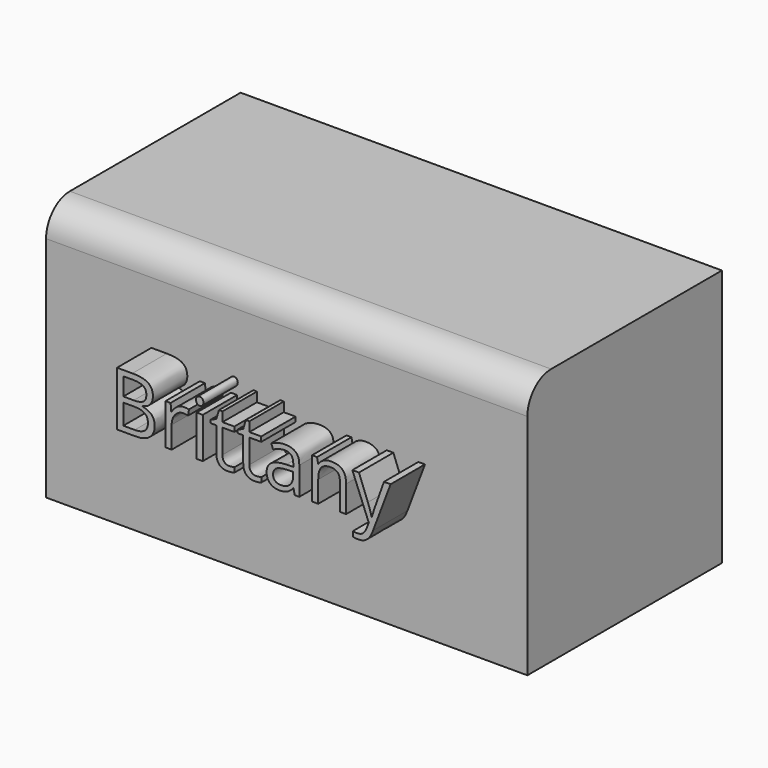
from build123d import *

# Parameters (mm, degrees)
F0_W         = 82.4485719204
F0_H         = 44.124007225
F1_DEPTH     = 41.656
F2_T         = -2.54
F3_R         = 5.08
F4_TEXT_SIZE = 13.0546641433
F5_DEPTH     = 49.022


# Not quite as in the source:
# - Text() gives the source's letters only with a copy of the font that has no kerning and outlines rounded to 1/6400 em; it was checked with that copy


with BuildPart() as f1:
    # F0 (on Front) → F1 (new body)
    with BuildSketch(Plane.XZ):
        with Locations((41.2242859602, 22.0620036125)):
            Rectangle(F0_W, F0_H)
    extrude(amount=F1_DEPTH)

    # F2
    f2_openings = [f1.faces().sort_by_distance(p)[0] for p in [
        (41.224286, -20.828, 0),
    ]]
    offset(amount=F2_T, openings=f2_openings)

    # F3
    f3_edges = [f1.edges().sort_by_distance(p)[0] for p in [
        (41.224286, -41.656, 44.124007),
    ]]
    fillet(f3_edges, radius=F3_R)

    # F4 (on Front) → F5 (join)
    with BuildSketch(Plane.XZ):
        with Locations((16.7637001723, 19.1239435226)):
            Text('Brittany', F4_TEXT_SIZE, font='Open Sans', text_align=(TextAlign.LEFT, TextAlign.BOTTOM))
    extrude(amount=F5_DEPTH)


solid = f1.part
